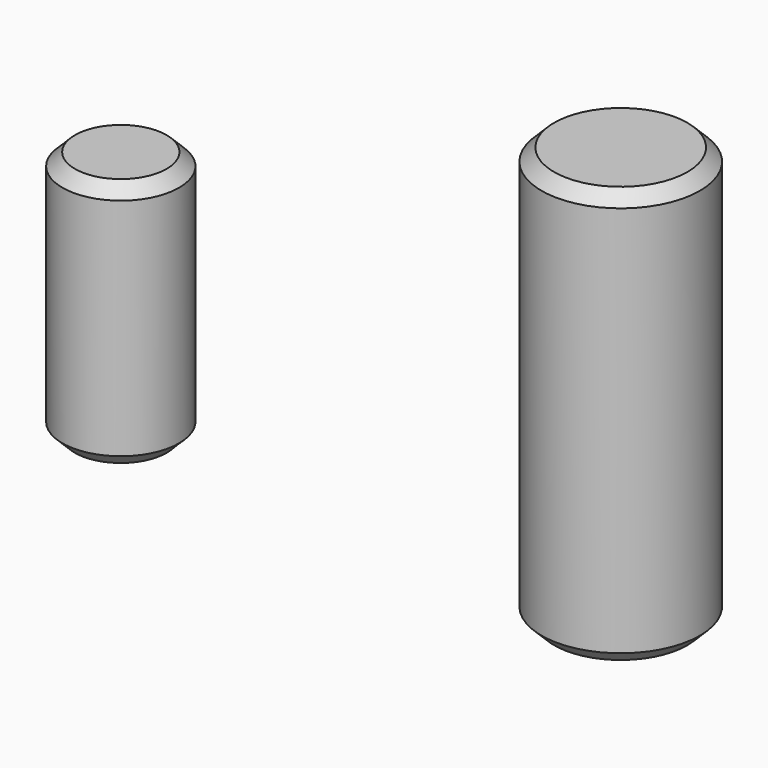
from build123d import *

# Parameters (mm, degrees)
F0_R      = 1.9
F1_DEPTH  = 10
F0_R_2    = 1.4
F2_DEPTH  = 6
F3_SIZE   = 0.3
F3_2_SIZE = 0.3


with BuildPart() as f1:
    # F0 (on Top) → F1 (new body)
    with BuildSketch(Plane.XY):
        with Locations((12, 0)):
            Circle(F0_R)
    extrude(amount=F1_DEPTH)

    # F3
    f3_edges = [f1.edges().sort_by_distance(p)[0] for p in [
        (10.1, 0, 10),
        (10.1, 0, 0),
    ]]
    chamfer(f3_edges, length=F3_SIZE)


with BuildPart() as f2:
    # F0 (on Top) → F2 (new body)
    with BuildSketch(Plane.XY):
        Circle(F0_R_2)
    extrude(amount=F2_DEPTH)

    # F3#2
    f3_2_edges = [f2.edges().sort_by_distance(p)[0] for p in [
        (-1.4, 0, 6),
        (-1.4, 0, 0),
    ]]
    chamfer(f3_2_edges, length=F3_2_SIZE)


solid = Compound([f1.part, f2.part])
